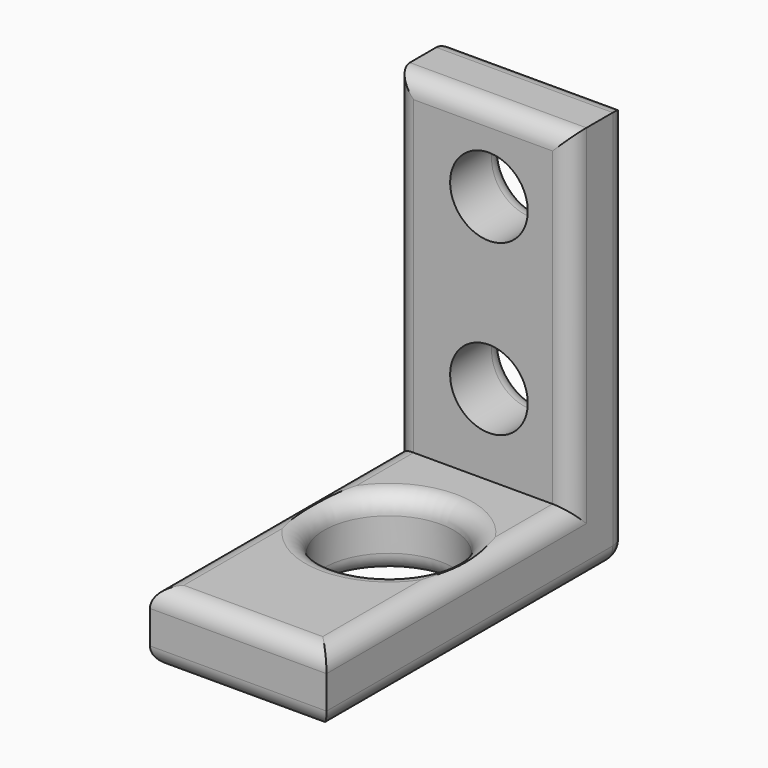
from build123d import *

# Parameters (mm, degrees)
F1_W         = 7.5
F1_H         = 3
F2_DEPTH     = 14
F0_W         = 7.5
F0_H         = 16
F0_R         = 2.75
F3_DEPTH     = 3
F4_R         = 1.65
F5_DEPTH     = 25
F6_T1_DEPTH  = 11.5
F6_T3_DEPTH  = 5.9
F6_T5_DEPTH  = 18.2
F6_T7_DEPTH  = 17.2
F6_T9_DEPTH  = 15
F6_T11_DEPTH = 16
F6_S15_W     = 0.8
F6_S15_H     = 0.8
F6_T16_DEPTH = 0.8
F6_S21_W     = 0.8
F6_S21_H     = 0.8
F6_T22_DEPTH = 0.8
F6_T37_DEPTH = 18
F6_T41_DEPTH = 17
F6_T48_DEPTH = 18
F6_T52_DEPTH = 17


# Not quite as in the source:
# - a fillet or chamfer that OpenCascade refuses, or shapes differently, is made with other operations: its cross-section is extruded or revolved along the edge and cut away or added


with BuildPart() as f2:
    # F1 (on face) → F2 (new body)
    with BuildSketch(Plane.XY):
        with Locations((3.75, 14.5)):
            Rectangle(F1_W, F1_H)
    extrude(amount=F2_DEPTH)

    # F0 (on Top) → F3 (join)
    with BuildSketch(Plane.XY):
        with Locations((3.75, 8)):
            Rectangle(F0_W, F0_H)
        with Locations((3.75, 8)):
            Circle(F0_R, mode=Mode.SUBTRACT)
    extrude(amount=-F3_DEPTH)

    # F4 (on face) → F5 (cut)
    with BuildSketch(Plane(origin=(0, 16, 0), x_dir=(-1, 0, 0), z_dir=(0, 1, 0))):
        with Locations((-4, 3.4267012961)):
            Circle(F4_R)
        with Locations((-4, 10.6111699715)):
            Circle(F4_R)
    extrude(amount=-F5_DEPTH, mode=Mode.SUBTRACT)

    # F6: fillet of radius 0.8 on 17 edges, made by hand

    # F6_s2 → F6_t1 (cut)
    with BuildSketch(Plane.YZ.offset(-2)):
        with BuildLine():
            ThreePointArc((16, 13.2), (15.7656854249, 13.7656854249), (15.2, 14))
            Line((15.2, 14), (16, 14))
            Line((16, 14), (16, 13.2))
        make_face()
        with BuildLine():
            ThreePointArc((13.8, 14), (13.2343145751, 13.7656854249), (13, 13.2))
            Line((13, 13.2), (13, 14))
            Line((13, 14), (13.8, 14))
        make_face()
        with BuildLine():
            ThreePointArc((0.8, 0), (0.2343145751, -0.2343145751), (0, -0.8))
            Line((0, -0.8), (0, 0))
            Line((0, 0), (0.8, 0))
        make_face()
        with BuildLine():
            ThreePointArc((0, -2.2), (0.2343145751, -2.7656854249), (0.8, -3))
            Line((0.8, -3), (0, -3))
            Line((0, -3), (0, -2.2))
        make_face()
    extrude(amount=F6_T1_DEPTH, mode=Mode.SUBTRACT)

    # F6_s4 → F6_t3 (cut)
    with BuildSketch(Plane.YZ.offset(0.8)):
        with BuildLine():
            ThreePointArc((16, -2.2), (15.7656854249, -2.7656854249), (15.2, -3))
            Line((15.2, -3), (16, -3))
            Line((16, -3), (16, -2.2))
        make_face()
    extrude(amount=F6_T3_DEPTH, mode=Mode.SUBTRACT)

    # F6_s6 → F6_t5 (cut)
    with BuildSketch(Plane.XY.offset(-2.2)):
        with BuildLine():
            ThreePointArc((0, 15.2), (0.2343145751, 15.7656854249), (0.8, 16))
            Line((0.8, 16), (0, 16))
            Line((0, 16), (0, 15.2))
        make_face()
        with BuildLine():
            ThreePointArc((6.7, 16), (7.2656854249, 15.7656854249), (7.5, 15.2))
            Line((7.5, 15.2), (7.5, 16))
            Line((7.5, 16), (6.7, 16))
        make_face()
    extrude(amount=F6_T5_DEPTH, mode=Mode.SUBTRACT)

    # F6_s8 → F6_t7 (cut)
    with BuildSketch(Plane.XZ.offset(-15.2)):
        with BuildLine():
            ThreePointArc((0, -2.2), (0.2343145751, -2.7656854249), (0.8, -3))
            Line((0.8, -3), (0, -3))
            Line((0, -3), (0, -2.2))
        make_face()
        with BuildLine():
            ThreePointArc((6.7, -3), (7.2656854249, -2.7656854249), (7.5, -2.2))
            Line((7.5, -2.2), (7.5, -3))
            Line((7.5, -3), (6.7, -3))
        make_face()
    extrude(amount=F6_T7_DEPTH, mode=Mode.SUBTRACT)

    # F6_s10 → F6_t9 (cut)
    with BuildSketch(Plane.XZ.offset(-13)):
        with BuildLine():
            ThreePointArc((0, -0.8), (0.2343145751, -0.2343145751), (0.8, 0))
            Line((0.8, 0), (0, 0))
            Line((0, 0), (0, -0.8))
        make_face()
        with BuildLine():
            ThreePointArc((6.7, 0), (7.2656854249, -0.2343145751), (7.5, -0.8))
            Line((7.5, -0.8), (7.5, 0))
            Line((7.5, 0), (6.7, 0))
        make_face()
    extrude(amount=F6_T9_DEPTH, mode=Mode.SUBTRACT)

    # F6_s12 → F6_t11 (cut)
    with BuildSketch(Plane.XY):
        with BuildLine():
            ThreePointArc((0, 13.8), (0.2343145751, 13.2343145751), (0.8, 13))
            Line((0.8, 13), (0, 13))
            Line((0, 13), (0, 13.8))
        make_face()
        with BuildLine():
            ThreePointArc((6.7, 13), (7.2656854249, 13.2343145751), (7.5, 13.8))
            Line((7.5, 13.8), (7.5, 13))
            Line((7.5, 13), (6.7, 13))
        make_face()
    extrude(amount=F6_T11_DEPTH, mode=Mode.SUBTRACT)


with BuildPart() as f6_tool14:
    # F6_s15 → F6_t16 (new body)
    with BuildSketch(Plane.XZ.offset(-15.2)):
        with Locations((7.1, -2.6)):
            Rectangle(F6_S15_W, F6_S15_H)
    extrude(amount=-F6_T16_DEPTH)

    # F6_s17 → F6_t18 (revolve, cut)
    with BuildSketch(Plane(origin=(6.7, 15.2, -2.2), x_dir=(-0.7071067812, 0, 0.7071067812), z_dir=(-0.7071067812, 0, -0.7071067812))):
        with BuildLine():
            ThreePointArc((0, -0.8), (0.8, 0), (0, 0.8))
            Line((0, 0.8), (0, -0.8))
        make_face()
    revolve(axis=Axis((6.7, 15.2, -2.2), (0, 1, 0)), mode=Mode.SUBTRACT)


with BuildPart() as f2_1:
    add(f2.part)

    # F6_t13: cut F6_tool14
    add(f6_tool14.part, mode=Mode.SUBTRACT)


with BuildPart() as f6_tool20:
    # F6_s21 → F6_t22 (new body)
    with BuildSketch(Plane.YZ.offset(0.8)):
        with Locations((15.6, -2.6)):
            Rectangle(F6_S21_W, F6_S21_H)
    extrude(amount=-F6_T22_DEPTH)

    # F6_s23 → F6_t24 (revolve, cut)
    with BuildSketch(Plane(origin=(0.8, 15.2, -2.2), x_dir=(0, -0.7071067812, 0.7071067812), z_dir=(0, -0.7071067812, -0.7071067812))):
        with BuildLine():
            ThreePointArc((0, -0.8), (0.8, 0), (0, 0.8))
            Line((0, 0.8), (0, -0.8))
        make_face()
    revolve(axis=Axis((0.8, 15.2, -2.2), (-1, 0, 0)), mode=Mode.SUBTRACT)


with BuildPart() as f2_2:
    add(f2_1.part)

    # F6_t19: cut F6_tool20
    add(f6_tool20.part, mode=Mode.SUBTRACT)

    # F6_s25 → F6_t26 (revolve, cut)
    with BuildSketch(Plane.XY.offset(10.6111699715)):
        with BuildLine():
            ThreePointArc((1.55, 16), (2.1156854249, 15.7656854249), (2.35, 15.2))
            Line((2.35, 15.2), (2.35, 16))
            Line((2.35, 16), (1.55, 16))
        make_face()
    revolve(axis=Axis((4, 16, 10.6111699715), (0, 1, 0)), mode=Mode.SUBTRACT)

    # F6_s27 → F6_t28 (revolve, cut)
    with BuildSketch(Plane.XY.offset(3.4267012961)):
        with BuildLine():
            ThreePointArc((1.55, 16), (2.1156854249, 15.7656854249), (2.35, 15.2))
            Line((2.35, 15.2), (2.35, 16))
            Line((2.35, 16), (1.55, 16))
        make_face()
    revolve(axis=Axis((4, 16, 3.4267012961), (0, 1, 0)), mode=Mode.SUBTRACT)

    # F6_s29 → F6_t30 (revolve, cut)
    with BuildSketch(Plane.XZ.offset(-8)):
        with BuildLine():
            ThreePointArc((7.3, -3), (6.7343145751, -2.7656854249), (6.5, -2.2))
            Line((6.5, -2.2), (6.5, -3))
            Line((6.5, -3), (7.3, -3))
        make_face()
    revolve(axis=Axis((3.75, 8, -3), (0, 0, 1)), mode=Mode.SUBTRACT)

    # F6_s31 → F6_t32 (revolve, cut)
    with BuildSketch(Plane.XZ.offset(-8)):
        with BuildLine():
            ThreePointArc((7.3, 0), (6.7343145751, -0.2343145751), (6.5, -0.8))
            Line((6.5, -0.8), (6.5, 0))
            Line((6.5, 0), (7.3, 0))
        make_face()
    revolve(axis=Axis((3.75, 8, 0), (0, 0, 1)), mode=Mode.SUBTRACT)


with BuildPart() as f6_tool35:
    # F6_s36 → F6_t37 (new body)
    with BuildSketch(Plane.XY.offset(-2)):
        with BuildLine():
            ThreePointArc((0, 13.8), (0.2343145751, 13.2343145751), (0.8, 13))
            Line((0.8, 13), (0, 13))
            Line((0, 13), (0, 13.8))
        make_face()
    extrude(amount=F6_T37_DEPTH)

    split(bisect_by=Plane.XY, keep=Keep.BOTTOM)


with BuildPart() as f6_tool39:
    # F6_s40 → F6_t41 (new body)
    with BuildSketch(Plane.XZ.offset(-15)):
        with BuildLine():
            ThreePointArc((0, -0.8), (0.2343145751, -0.2343145751), (0.8, 0))
            Line((0.8, 0), (0, 0))
            Line((0, 0), (0, -0.8))
        make_face()
    extrude(amount=F6_T41_DEPTH)

    split(bisect_by=Plane.XZ.offset(-13), keep=Keep.BOTTOM)


with BuildPart() as f6_tool35_1:
    add(f6_tool35.part)

    # F6_t43: intersect F6_tool39
    add(f6_tool39.part, mode=Mode.INTERSECT)


with BuildPart() as f2_3:
    add(f2_2.part)

    # F6_t33: cut F6_tool35
    add(f6_tool35_1.part, mode=Mode.SUBTRACT)


with BuildPart() as f6_tool46:
    # F6_s47 → F6_t48 (new body)
    with BuildSketch(Plane.XY.offset(-2)):
        with BuildLine():
            ThreePointArc((6.7, 13), (7.2656854249, 13.2343145751), (7.5, 13.8))
            Line((7.5, 13.8), (7.5, 13))
            Line((7.5, 13), (6.7, 13))
        make_face()
    extrude(amount=F6_T48_DEPTH)

    split(bisect_by=Plane.XY, keep=Keep.BOTTOM)


with BuildPart() as f6_tool50:
    # F6_s51 → F6_t52 (new body)
    with BuildSketch(Plane.XZ.offset(2)):
        with BuildLine():
            ThreePointArc((6.7, 0), (7.2656854249, -0.2343145751), (7.5, -0.8))
            Line((7.5, -0.8), (7.5, 0))
            Line((7.5, 0), (6.7, 0))
        make_face()
    extrude(amount=-F6_T52_DEPTH)

    split(bisect_by=Plane.XZ.offset(-13), keep=Keep.BOTTOM)


with BuildPart() as f6_tool46_1:
    add(f6_tool46.part)

    # F6_t54: intersect F6_tool50
    add(f6_tool50.part, mode=Mode.INTERSECT)


with BuildPart() as f2_4:
    add(f2_3.part)

    # F6_t44: cut F6_tool46
    add(f6_tool46_1.part, mode=Mode.SUBTRACT)


solid = f2_4.part
